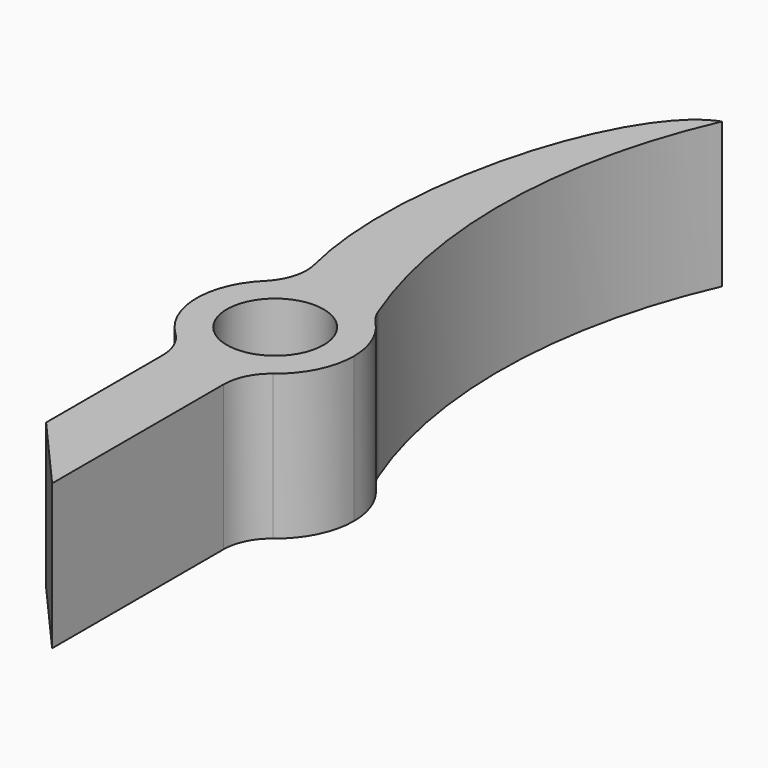
from build123d import *

# Parameters (mm, degrees)
F0_R     = 2
F1_DEPTH = 6
F2_R     = 2


# Not quite as in the source:
# - a feature names something its author has since deleted; it is built from what else it names


with BuildPart() as f1:
    # F0 (on Top) → F1 (new body)
    with BuildSketch(Plane.XY):
        with BuildLine():
            ThreePointArc((1.1986346156, -3.0208897792), (2.688685785, -1.8257789432), (3.25, 0))
            ThreePointArc((3.25, 0), (2.9473803034, 1.3694704624), (2.0958773247, 2.4839078565))
            ThreePointArc((2.0958773247, 2.4839078565), (0.4368938689, 3.220500543), (-1.3583713088, 2.952512047))
            ThreePointArc((-1.3583713088, 2.952512047), (-3.2469183887, 0.1414955013), (-1.6100655086, -2.8231523264))
            ThreePointArc((-1.6100655086, -2.8231523264), (-0.2282408158, -3.2419756523), (1.1986346156, -3.0208897792))
        make_face()
        Circle(F0_R, mode=Mode.SUBTRACT)
        with BuildLine():
            Line((1.1986346156, -13.0208897792), (1.1986346156, -3.0208897792))
            ThreePointArc((1.1986346156, -3.0208897792), (-0.2282408158, -3.2419756523), (-1.6100655086, -2.8231523264))
            Line((-1.6100655086, -2.8231523264), (-1.6100655086, -9.8231523264))
            Line((-1.6100655086, -9.8231523264), (1.1986346156, -13.0208897792))
        make_face()
        with BuildLine():
            ThreePointArc((-1.3583713088, 2.952512047), (0.4368938689, 3.220500543), (2.0958773247, 2.4839078565))
            ThreePointArc((2.0958773247, 2.4839078565), (0.3587431794, 11.3732693794), (2.2789172363, 20.2248971909))
            add(Edge.make_bspline(
                [(-1.3583713088, 2.952512047), (-3.6481465213, 9.1469325125), (-0.8962951833, 19.0959330648), (2.2789172363, 20.2248971909)],
                knots=[0, 0, 0, 0, 17.6512083587, 17.6512083587, 17.6512083587, 17.6512083587], degree=3))
        make_face()
    extrude(amount=F1_DEPTH)

    # F2
    f2_edges = [f1.edges().sort_by_distance(p)[0] for p in [
        (-1.610066, -2.823152, 3),
        (1.198635, -3.02089, 3),
        (-1.358371, 2.952512, 3),
        (2.095877, 2.483908, 3),
    ]]
    fillet(f2_edges, radius=F2_R)


solid = f1.part
